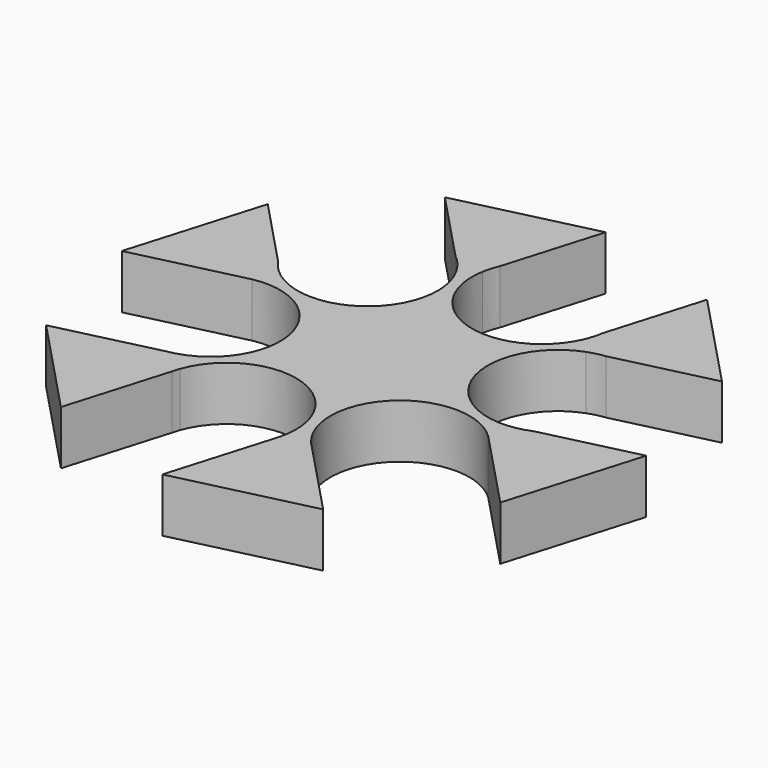
from build123d import *

# Parameters (mm, degrees)
F1_DEPTH = 10


# Not quite as in the source:
# - a feature of the source that left no trace in its solid (it failed there, or was rolled back) is left out


with BuildPart() as f1:
    # F0 (on Top) → F1 (new body)
    with BuildSketch(Plane.XY):
        with BuildLine():
            Line((-29.9939722279, 12.9722623931), (-42.3191245349, 25.9821456543))
            Line((-42.3191245349, 25.9821456543), (-49.6405097403, 1.341635914))
            Line((-49.6405097403, 1.341635914), (-29.3788570259, 6.1880200524))
            ThreePointArc((-29.3788570259, 6.1880200524), (-14.4470126823, -3.3975764275), (-23.2838200208, -18.7844042826))
            ThreePointArc((-23.2838200208, -18.7844042826), (-23.9549101464, -18.9642061938), (-24.6347260756, -19.1075274636))
            Line((-24.6347260756, -19.1075274636), (-43.6607604489, -23.658364086))
            Line((-43.6607604489, -23.658364086), (-25.9821456543, -42.3191245349))
            Line((-25.9821456543, -42.3191245349), (-20.4059776484, -23.5522357279))
            ThreePointArc((-20.4059776484, -23.5522357279), (-20.2283734176, -22.8904168158), (-20.0157770781, -22.2389950387))
            ThreePointArc((-20.0157770781, -22.2389950387), (-4.0233304879, -14.28870031), (4.4989162669, -29.9838219872))
            ThreePointArc((4.4989162669, -29.9838219872), (4.4318374321, -30.2176557723), (4.3603484872, -30.4501791902))
            Line((4.3603484872, -30.4501791902), (-1.341635914, -49.6405097403))
            Line((-1.341635914, -49.6405097403), (23.658364086, -43.6607604489))
            Line((23.658364086, -43.6607604489), (10.2042067758, -29.4591496596))
            ThreePointArc((10.2042067758, -29.4591496596), (9.7129486903, -28.9678695182), (9.2489208652, -28.4507922885))
            ThreePointArc((9.2489208652, -28.4507922885), (10.2477999291, -10.735096536), (27.9912063973, -10.8582317502))
            Line((27.9912063973, -10.8582317502), (42.3191245349, -25.9821456543))
            Line((42.3191245349, -25.9821456543), (49.6405097403, -1.341635914))
            Line((49.6405097403, -1.341635914), (32.2110441824, -5.5105892868))
            ThreePointArc((32.2110441824, -5.5105892868), (30.1080602508, -6.2077620929), (27.9172204019, -6.5376288751))
            ThreePointArc((27.9172204019, -6.5376288751), (14.3772643763, 3.7032958994), (22.517444526, 18.6010949497))
            ThreePointArc((22.517444526, 18.6010949497), (24.0610630231, 19.0733865517), (25.6513214754, 19.3506868884))
            Line((25.6513214754, 19.3506868884), (43.6607604489, 23.658364086))
            Line((43.6607604489, 23.658364086), (25.9821456543, 42.3191245349))
            Line((25.9821456543, 42.3191245349), (20.7505372467, 24.7118693081))
            ThreePointArc((20.7505372467, 24.7118693081), (20.3589951368, 22.9556577497), (19.7280350427, 21.2705839763))
            ThreePointArc((19.7280350427, 21.2705839763), (4.1315999448, 14.2550710192), (-4.8477844397, 28.8096876713))
            ThreePointArc((-4.8477844397, 28.8096876713), (-4.4924498123, 30.3397177103), (-3.9546627515, 31.8155360239))
            Line((-3.9546627515, 31.8155360239), (1.341635914, 49.6405097403))
            Line((1.341635914, 49.6405097403), (-23.658364086, 43.6607604489))
            Line((-23.658364086, 43.6607604489), (-10.9230867149, 30.2179673888))
            ThreePointArc((-10.9230867149, 30.2179673888), (-9.7422609409, 29.1173003575), (-8.7069825787, 27.8787463076))
            ThreePointArc((-8.7069825787, 27.8787463076), (-10.0224304809, 10.9531282619), (-26.9576179635, 9.767221714))
            ThreePointArc((-26.9576179635, 9.767221714), (-28.6128792901, 11.2398728194), (-29.9939722279, 12.9722623931))
        make_face()
    extrude(amount=F1_DEPTH)


solid = f1.part
